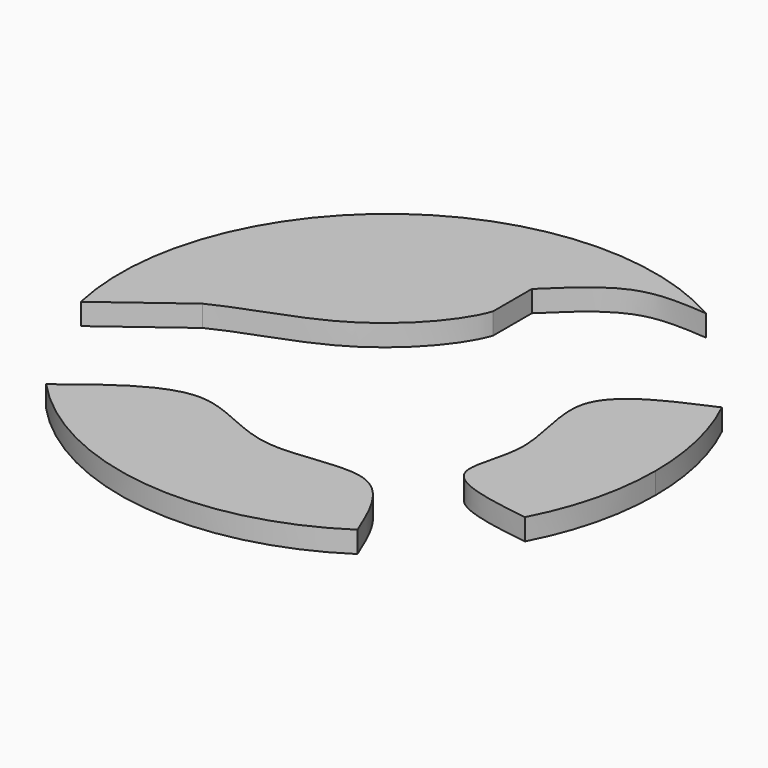
from build123d import *

# Parameters (mm, degrees)
F1_DEPTH = 2


with BuildPart() as f1:
    # F0 (on Top) → F1 (new body)
    with BuildSketch(Plane.XY):
        with BuildLine():
            ThreePointArc((22.1188925873, -11.6513772023), (24.2690370089, -6.001153444), (25, 0))
            ThreePointArc((25, 0), (24.3701069704, 5.5765478793), (22.5121691, 10.8720854676))
            add(Edge.make_bspline(
                [(22.5121691, 10.8720854676), (18.8895611428, 9.3055197167), (11.9102659407, 6.2896821538), (16.4364178682, -3.0658471403), (12.2521680449, -10.2063529762), (18.6615851191, -11.1474987265), (22.1188925873, -11.6513772023)],
                knots=[0, 0, 0, 0, 0.2780136343, 0.5343531988, 0.7479805585, 1, 1, 1, 1], degree=3))
        make_face()
    extrude(amount=F1_DEPTH)


with BuildPart() as f1b:
    # F0 (on Top) → F1, piece 2 (new body)
    with BuildSketch(Plane.XY):
        with BuildLine():
            add(Edge.make_bspline(
                [(0, 16.8172493577), (1.9144161531, 18.6824676113), (5.5934798745, 22.2645311542), (10.1584208321, 21.9120162799), (12.34633467, 21.7386296766)],
                knots=[0, 0, 0, 0, 0.5203475383, 1, 1, 1, 1], degree=3))
            ThreePointArc((12.34633467, 21.7386296766), (-14.8165901958, 20.1362522573), (-24.4273769181, -5.3200805351))
            add(Edge.make_bspline(
                [(-24.4273769181, -5.3200805351), (-22.2453911763, -3.3574319676), (-20.0634054345, -1.3947834001), (-17.3023622483, 0)],
                knots=[0, 0, 0, 0, 0.254891956, 0.254891956, 0.254891956, 0.254891956], degree=3))
            add(Edge.make_bspline(
                [(-17.3023622483, 0), (-14.1903788127, 1.5720662607), (-6.6472654424, 3.2397841474), (-0.8648455283, 9.7284013886), (0, 12.2895278037)],
                knots=[0.254891956, 0.254891956, 0.254891956, 0.254891956, 0.542181756, 0.8181160828, 0.8181160828, 0.8181160828, 0.8181160828], degree=3))
            Line((0, 12.2895278037), (0, 16.8172493577))
        make_face()
        with BuildLine():
            add(Edge.make_bspline(
                [(-24.4273769181, -5.3200805351), (-22.2453911763, -3.3574319676), (-20.0634054345, -1.3947834001), (-17.3023622483, 0)],
                knots=[0, 0, 0, 0, 0.254891956, 0.254891956, 0.254891956, 0.254891956], degree=3))
            Line((-24.4273769181, -5.3200805351), (-17.3023622483, 0))
        make_face()
    extrude(amount=F1_DEPTH)


with BuildPart() as f1c:
    # F0 (on Top) → F1, piece 3 (new body)
    with BuildSketch(Plane.XY):
        with BuildLine():
            ThreePointArc((-18.2737018092, -17.0608271249), (-2.9135456355, -24.8296446175), (13.8278126154, -20.8276642539))
            add(Edge.make_bspline(
                [(-18.2737018092, -17.0608271249), (-14.8332101277, -14.3400323801), (-8.3808524987, -9.228978734), (-0.4412585546, -15.998889193), (10.2263751779, -12.0238586347), (12.6576888155, -17.9664290501), (13.8278126154, -20.8276642539)],
                knots=[0, 0, 0, 0, 0.2769679297, 0.5181649262, 0.767240907, 1, 1, 1, 1], degree=3))
        make_face()
    extrude(amount=F1_DEPTH)


solid = Compound([f1.part, f1b.part, f1c.part])
